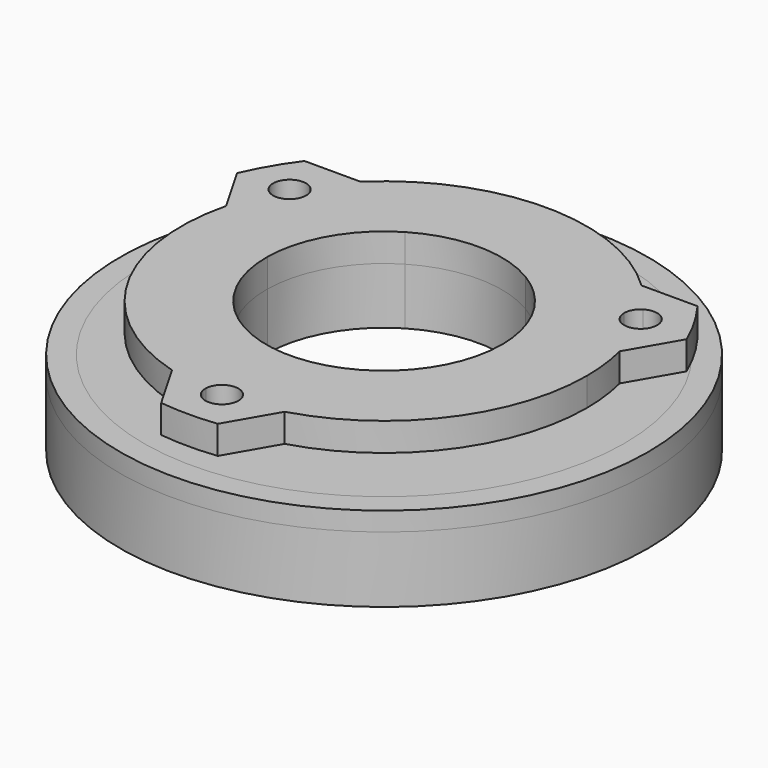
from build123d import *

# Parameters (mm, degrees)
F0_R          = 8.75
F0_R_2        = 7.75
F1_DEPTH      = 2
F0_R_3        = 12.75
F2_DEPTH      = 1
F0_R_4        = 14
F3_DEPTH      = 3.5
F3_DEPTH_BACK = 1
F5_DEPTH      = 1.5
F6_DEPTH      = 3


# Not quite as in the source:
# - ends of sketch curves that miss each other by under 0.0002 mm in the source are joined


with BuildPart() as f1:
    # F0 (on Top) → F1 (new body)
    with BuildSketch(Plane.XY):
        Circle(F0_R)
        Circle(F0_R_2, mode=Mode.SUBTRACT)
    extrude(amount=F1_DEPTH)

    # F0 (on Top) → F2 (join)
    with BuildSketch(Plane.XY):
        Circle(F0_R_3)
        Circle(F0_R, mode=Mode.SUBTRACT)
    extrude(amount=F2_DEPTH)

    # F0 (on Top) → F3 (join, two sides)
    with BuildSketch(Plane.XY) as f3_sk:
        Circle(F0_R_4)
        Circle(F0_R_3, mode=Mode.SUBTRACT)
    extrude(amount=-F3_DEPTH)
    extrude(f3_sk.sketch, amount=F3_DEPTH_BACK)


with BuildPart() as f5:
    # F4 (on face) → F5 (new body)
    with BuildSketch(Plane.XY.offset(2)):
        with BuildLine():
            Line((-7.4498323446, 7.7499998733), (-10.4241976301, 7.7499998733))
            ThreePointArc((-10.4241976301, 7.7499998733), (-11.2492131147, 6.49473622), (-11.9237955847, 5.1526200251))
            Line((-11.9237955847, 5.1526200251), (-10.436612942, 2.5767441277))
            ThreePointArc((-10.436612942, 2.5767441277), (-10.1269990673, 3.606437285), (-9.7160710573, 4.6000503485))
            ThreePointArc((-9.7160710573, 4.6000503485), (-10.067545319, 5.8125), (-8.8417959892, 6.1143391863))
            ThreePointArc((-8.8417959892, 6.1143391863), (-8.1867658396, 6.9670198139), (-7.4498323446, 7.7499998733))
        make_face()
        with BuildLine():
            Line((1.4995979546, -12.9026198984), (2.9867805973, -10.3267440011))
            ThreePointArc((2.9867805973, -10.3267440011), (1.9402332277, -10.5734570989), (0.8742750681, -10.7143895349))
            ThreePointArc((0.8742750681, -10.7143895349), (0.8748187483, -10.7321910784), (0.875, -10.75))
            ThreePointArc((0.875, -10.75), (-0.0178089216, -11.6248187483), (-0.8742750681, -10.7143895349))
            ThreePointArc((-0.8742750681, -10.7143895349), (-1.9402332277, -10.5734570989), (-2.9867805973, -10.3267440011))
            Line((-2.9867805973, -10.3267440011), (-1.4995979546, -12.9026198984))
            ThreePointArc((-1.4995979546, -12.9026198984), (0, -12.9894724399), (1.4995979546, -12.9026198984))
        make_face()
        with BuildLine():
            ThreePointArc((9.7160710573, 4.6000503485), (10.1269990673, 3.606437285), (10.436612942, 2.5767441277))
            Line((10.436612942, 2.5767441277), (11.9237955847, 5.1526200251))
            ThreePointArc((11.9237955847, 5.1526200251), (11.2492131147, 6.49473622), (10.4241976301, 7.7499998733))
            Line((10.4241976301, 7.7499998733), (7.4498323446, 7.7499998733))
            ThreePointArc((7.4498323446, 7.7499998733), (8.1867658396, 6.9670198139), (8.8417959892, 6.1143391863))
            ThreePointArc((8.8417959892, 6.1143391863), (9.7317594863, 6.1415197205), (10.1847730907, 5.375))
            ThreePointArc((10.1847730907, 5.375), (10.0584838896, 4.9221676474), (9.7160710573, 4.6000503485))
        make_face()
        with BuildLine():
            Line((4.062019444, 7.7499998733), (7.4498323446, 7.7499998733))
            ThreePointArc((7.4498323446, 7.7499998733), (0, 10.75), (-7.4498323446, 7.7499998733))
            Line((-7.4498323446, 7.7499998733), (-4.062019444, 7.7499998733))
            ThreePointArc((-4.062019444, 7.7499998733), (0, 8.75), (4.062019444, 7.7499998733))
        make_face()
        with BuildLine():
            Line((-4.062019444, 7.7499998733), (-7.4498323446, 7.7499998733))
            ThreePointArc((-7.4498323446, 7.7499998733), (-8.1867658396, 6.9670198139), (-8.8417959892, 6.1143391863))
            ThreePointArc((-8.8417959892, 6.1143391863), (-8.5432533702, 5.7969863956), (-8.4347730907, 5.375))
            Line((-8.4347730907, 5.375), (-6.9044822398, 5.375))
            ThreePointArc((-6.9044822398, 5.375), (-5.6103650411, 6.7146335794), (-4.062019444, 7.7499998733))
        make_face()
        with BuildLine():
            Line((-6.9044822398, 5.375), (-8.4347730907, 5.375))
            ThreePointArc((-8.4347730907, 5.375), (-8.5520008624, 4.9375), (-8.8722730907, 4.6172277717))
            Line((-8.8722730907, 4.6172277717), (-8.1071276653, 3.2919570197))
            ThreePointArc((-8.1071276653, 3.2919570197), (-7.5777222831, 4.375), (-6.9044822398, 5.375))
        make_face()
        with BuildLine():
            ThreePointArc((-9.7160710573, 4.6000503485), (-10.1269990673, 3.606437285), (-10.436612942, 2.5767441277))
            Line((-10.436612942, 2.5767441277), (-8.7427064916, -0.3571879075))
            ThreePointArc((-8.7427064916, -0.3571879075), (-8.6202257774, 1.5014018604), (-8.1071276653, 3.2919570197))
            Line((-8.1071276653, 3.2919570197), (-8.8722730907, 4.6172277717))
            ThreePointArc((-8.8722730907, 4.6172277717), (-9.2919641691, 4.5001812517), (-9.7160710573, 4.6000503485))
        make_face()
        with BuildLine():
            ThreePointArc((-10.436612942, 2.5767441277), (-9.3097730907, -5.375), (-2.9867805973, -10.3267440011))
            Line((-2.9867805973, -10.3267440011), (-4.6806870477, -7.3928119658))
            ThreePointArc((-4.6806870477, -7.3928119658), (-7.5777222831, -4.375), (-8.7427064916, -0.3571879075))
            Line((-8.7427064916, -0.3571879075), (-10.436612942, 2.5767441277))
        make_face()
        with BuildLine():
            ThreePointArc((-2.9867805973, -10.3267440011), (-1.9402332277, -10.5734570989), (-0.8742750681, -10.7143895349))
            ThreePointArc((-0.8742750681, -10.7143895349), (-0.7487107989, -10.2971676474), (-0.4375, -9.9922277717))
            Line((-0.4375, -9.9922277717), (-1.2026454254, -8.6669570197))
            ThreePointArc((-1.2026454254, -8.6669570197), (-3.0098607363, -8.2160354398), (-4.6806870477, -7.3928119658))
            Line((-4.6806870477, -7.3928119658), (-2.9867805973, -10.3267440011))
        make_face()
        with BuildLine():
            ThreePointArc((0.8742750681, -10.7143895349), (1.9402332277, -10.5734570989), (2.9867805973, -10.3267440011))
            Line((2.9867805973, -10.3267440011), (4.6806870477, -7.3928119658))
            ThreePointArc((4.6806870477, -7.3928119658), (3.0098607363, -8.2160354398), (1.2026454254, -8.6669570197))
            Line((1.2026454254, -8.6669570197), (0.4375, -9.9922277717))
            ThreePointArc((0.4375, -9.9922277717), (0.7487107989, -10.2971676474), (0.8742750681, -10.7143895349))
        make_face()
        with BuildLine():
            ThreePointArc((2.9867805973, -10.3267440011), (8.592740873, -6.4596675061), (10.75, 0))
            ThreePointArc((10.75, 0), (10.6713656372, 1.2978657238), (10.436612942, 2.5767441277))
            Line((10.436612942, 2.5767441277), (8.7427064916, -0.3571879075))
            ThreePointArc((8.7427064916, -0.3571879075), (7.5777222831, -4.375), (4.6806870477, -7.3928119658))
            Line((4.6806870477, -7.3928119658), (2.9867805973, -10.3267440011))
        make_face()
        with BuildLine():
            Line((8.7427064916, -0.3571879075), (10.436612942, 2.5767441277))
            ThreePointArc((10.436612942, 2.5767441277), (10.1269990673, 3.606437285), (9.7160710573, 4.6000503485))
            ThreePointArc((9.7160710573, 4.6000503485), (9.2919641691, 4.5001812517), (8.8722730907, 4.6172277717))
            Line((8.8722730907, 4.6172277717), (8.1071276653, 3.2919570197))
            ThreePointArc((8.1071276653, 3.2919570197), (8.5877781489, 1.6770707989), (8.75, 0))
            ThreePointArc((8.75, 0), (8.7481764329, -0.1786311819), (8.7427064916, -0.3571879075))
        make_face()
        with BuildLine():
            Line((8.1071276653, 3.2919570197), (8.8722730907, 4.6172277717))
            ThreePointArc((8.8722730907, 4.6172277717), (8.5520008624, 4.9375), (8.4347730907, 5.375))
            Line((8.4347730907, 5.375), (6.9044822398, 5.375))
            ThreePointArc((6.9044822398, 5.375), (7.5777222831, 4.375), (8.1071276653, 3.2919570197))
        make_face()
        with BuildLine():
            ThreePointArc((8.4347730907, 5.375), (8.5432533702, 5.7969863956), (8.8417959892, 6.1143391863))
            ThreePointArc((8.8417959892, 6.1143391863), (8.1867658396, 6.9670198139), (7.4498323446, 7.7499998733))
            Line((7.4498323446, 7.7499998733), (4.062019444, 7.7499998733))
            ThreePointArc((4.062019444, 7.7499998733), (5.6103650411, 6.7146335794), (6.9044822398, 5.375))
            Line((6.9044822398, 5.375), (8.4347730907, 5.375))
        make_face()
        with BuildLine():
            ThreePointArc((-0.4375, -9.9922277717), (0, -9.875), (0.4375, -9.9922277717))
            Line((0.4375, -9.9922277717), (1.2026454254, -8.6669570197))
            ThreePointArc((1.2026454254, -8.6669570197), (0, -8.75), (-1.2026454254, -8.6669570197))
            Line((-1.2026454254, -8.6669570197), (-0.4375, -9.9922277717))
        make_face()
        with BuildLine():
            Line((0, 7.7499998733), (4.062019444, 7.7499998733))
            ThreePointArc((4.062019444, 7.7499998733), (0, 8.75), (-4.062019444, 7.7499998733))
            Line((-4.062019444, 7.7499998733), (0, 7.7499998733))
        make_face()
        with BuildLine():
            Line((0, 7.7499998733), (-4.062019444, 7.7499998733))
            ThreePointArc((-4.062019444, 7.7499998733), (-5.6103650411, 6.7146335794), (-6.9044822398, 5.375))
            Line((-6.9044822398, 5.375), (-5.5831778585, 5.375))
            ThreePointArc((-5.5831778585, 5.375), (-3.0336652749, 7.1315759128), (0, 7.7499998733))
        make_face()
        with BuildLine():
            Line((-5.5831778585, 5.375), (-6.9044822398, 5.375))
            ThreePointArc((-6.9044822398, 5.375), (-7.5777222831, 4.375), (-8.1071276653, 3.2919570197))
            Line((-8.1071276653, 3.2919570197), (-7.4464754746, 2.1476738593))
            ThreePointArc((-7.4464754746, 2.1476738593), (-6.7116968793, 3.875), (-5.5831778585, 5.375))
        make_face()
        with BuildLine():
            Line((-8.7427064916, -0.3571879075), (-6.7116967696, -3.8749999367))
            ThreePointArc((-6.7116967696, -3.8749999367), (-7.6929585469, -0.9385567618), (-7.4464754746, 2.1476738593))
            Line((-7.4464754746, 2.1476738593), (-8.1071276653, 3.2919570197))
            ThreePointArc((-8.1071276653, 3.2919570197), (-8.6202257774, 1.5014018604), (-8.7427064916, -0.3571879075))
        make_face()
        with BuildLine():
            ThreePointArc((-8.7427064916, -0.3571879075), (-7.5777222831, -4.375), (-4.6806870477, -7.3928119658))
            Line((-4.6806870477, -7.3928119658), (-6.7116967696, -3.8749999367))
            Line((-6.7116967696, -3.8749999367), (-8.7427064916, -0.3571879075))
        make_face()
        with BuildLine():
            ThreePointArc((-4.6806870477, -7.3928119658), (-3.0098607363, -8.2160354398), (-1.2026454254, -8.6669570197))
            Line((-1.2026454254, -8.6669570197), (-1.8632976161, -7.5226738593))
            ThreePointArc((-1.8632976161, -7.5226738593), (-4.6592932721, -6.193019151), (-6.7116968793, -3.875))
            Line((-6.7116968793, -3.875), (-4.6806870477, -7.3928119658))
        make_face()
        with BuildLine():
            ThreePointArc((-1.2026454254, -8.6669570197), (0, -8.75), (1.2026454254, -8.6669570197))
            Line((1.2026454254, -8.6669570197), (1.8632976161, -7.5226738593))
            ThreePointArc((1.8632976161, -7.5226738593), (0, -7.75), (-1.8632976161, -7.5226738593))
            Line((-1.8632976161, -7.5226738593), (-1.2026454254, -8.6669570197))
        make_face()
        with BuildLine():
            ThreePointArc((1.2026454254, -8.6669570197), (3.0098607363, -8.2160354398), (4.6806870477, -7.3928119658))
            Line((4.6806870477, -7.3928119658), (6.7116967696, -3.8749999367))
            ThreePointArc((6.7116967696, -3.8749999367), (4.6592932721, -6.193019151), (1.8632976161, -7.5226738593))
            Line((1.8632976161, -7.5226738593), (1.2026454254, -8.6669570197))
        make_face()
        with BuildLine():
            ThreePointArc((4.6806870477, -7.3928119658), (7.5777222831, -4.375), (8.7427064916, -0.3571879075))
            Line((8.7427064916, -0.3571879075), (6.7116967696, -3.8749999367))
            Line((6.7116967696, -3.8749999367), (4.6806870477, -7.3928119658))
        make_face()
        with BuildLine():
            Line((6.7116967696, -3.8749999367), (8.7427064916, -0.3571879075))
            ThreePointArc((8.7427064916, -0.3571879075), (8.7481764329, -0.1786311819), (8.75, 0))
            ThreePointArc((8.75, 0), (8.5877781489, 1.6770707989), (8.1071276653, 3.2919570197))
            Line((8.1071276653, 3.2919570197), (7.4464754746, 2.1476738593))
            ThreePointArc((7.4464754746, 2.1476738593), (7.6737437059, 1.0845079695), (7.75, 0))
            ThreePointArc((7.75, 0), (7.4859251537, -2.0058475995), (6.7116967696, -3.8749999367))
        make_face()
        with BuildLine():
            Line((7.4464754746, 2.1476738593), (8.1071276653, 3.2919570197))
            ThreePointArc((8.1071276653, 3.2919570197), (7.5777222831, 4.375), (6.9044822398, 5.375))
            Line((6.9044822398, 5.375), (5.5831778585, 5.375))
            ThreePointArc((5.5831778585, 5.375), (6.7116968793, 3.875), (7.4464754746, 2.1476738593))
        make_face()
        with BuildLine():
            Line((5.5831778585, 5.375), (6.9044822398, 5.375))
            ThreePointArc((6.9044822398, 5.375), (5.6103650411, 6.7146335794), (4.062019444, 7.7499998733))
            Line((4.062019444, 7.7499998733), (0, 7.7499998733))
            ThreePointArc((0, 7.7499998733), (3.0336652749, 7.1315759128), (5.5831778585, 5.375))
        make_face()
        with BuildLine():
            Line((3.1893377055, 5.375), (5.5831778585, 5.375))
            ThreePointArc((5.5831778585, 5.375), (3.0336652749, 7.1315759128), (0, 7.75))
            ThreePointArc((0, 7.75), (-3.0336652749, 7.1315759128), (-5.5831778585, 5.375))
            Line((-5.5831778585, 5.375), (-3.1893377055, 5.375))
            ThreePointArc((-3.1893377055, 5.375), (0, 6.25), (3.1893377055, 5.375))
        make_face()
        with BuildLine():
            Line((-3.1893377055, 5.375), (-5.5831778585, 5.375))
            ThreePointArc((-5.5831778585, 5.375), (-6.7116968793, 3.875), (-7.4464754746, 2.1476738593))
            Line((-7.4464754746, 2.1476738593), (-6.2495553981, 0.0745474742))
            ThreePointArc((-6.2495553981, 0.0745474742), (-5.4126587737, 3.125), (-3.1893377055, 5.375))
        make_face()
        with BuildLine():
            ThreePointArc((-6.7116968793, -3.875), (-4.6592932721, -6.193019151), (-1.8632976161, -7.5226738593))
            Line((-1.8632976161, -7.5226738593), (-3.0602176926, -5.4495474742))
            ThreePointArc((-3.0602176926, -5.4495474742), (-5.4126587737, -3.125), (-6.2495553981, 0.0745474742))
            Line((-6.2495553981, 0.0745474742), (-7.4464754746, 2.1476738593))
            ThreePointArc((-7.4464754746, 2.1476738593), (-7.6929585469, -0.9385567618), (-6.7116968793, -3.875))
        make_face()
        with BuildLine():
            ThreePointArc((1.8632976161, -7.5226738593), (4.6592932721, -6.193019151), (6.7116968793, -3.875))
            ThreePointArc((6.7116968793, -3.875), (7.4859251537, -2.0058475995), (7.75, 0))
            ThreePointArc((7.75, 0), (7.6737437059, 1.0845079695), (7.4464754746, 2.1476738593))
            Line((7.4464754746, 2.1476738593), (6.2495553981, 0.0745474742))
            ThreePointArc((6.2495553981, 0.0745474742), (6.2498888485, 0.0372744), (6.25, 0))
            ThreePointArc((6.25, 0), (5.3939253137, -3.1572250016), (3.0602176926, -5.4495474742))
            Line((3.0602176926, -5.4495474742), (1.8632976161, -7.5226738593))
        make_face()
        with BuildLine():
            Line((6.2495553981, 0.0745474742), (7.4464754746, 2.1476738593))
            ThreePointArc((7.4464754746, 2.1476738593), (6.7116968793, 3.875), (5.5831778585, 5.375))
            Line((5.5831778585, 5.375), (3.1893377055, 5.375))
            ThreePointArc((3.1893377055, 5.375), (5.4126587737, 3.125), (6.2495553981, 0.0745474742))
        make_face()
        with BuildLine():
            ThreePointArc((-1.8632976161, -7.5226738593), (0, -7.75), (1.8632976161, -7.5226738593))
            Line((1.8632976161, -7.5226738593), (3.0602176926, -5.4495474742))
            ThreePointArc((3.0602176926, -5.4495474742), (0, -6.25), (-3.0602176926, -5.4495474742))
            Line((-3.0602176926, -5.4495474742), (-1.8632976161, -7.5226738593))
        make_face()
    extrude(amount=F5_DEPTH)

    # F4 (on face) → F6 (join)
    with BuildSketch(Plane.XY.offset(2)):
        with BuildLine():
            Line((3.1893377055, 5.375), (5.5831778585, 5.375))
            ThreePointArc((5.5831778585, 5.375), (3.0336652749, 7.1315759128), (0, 7.75))
            ThreePointArc((0, 7.75), (-3.0336652749, 7.1315759128), (-5.5831778585, 5.375))
            Line((-5.5831778585, 5.375), (-3.1893377055, 5.375))
            ThreePointArc((-3.1893377055, 5.375), (0, 6.25), (3.1893377055, 5.375))
        make_face()
        with BuildLine():
            Line((-3.1893377055, 5.375), (-5.5831778585, 5.375))
            ThreePointArc((-5.5831778585, 5.375), (-6.7116968793, 3.875), (-7.4464754746, 2.1476738593))
            Line((-7.4464754746, 2.1476738593), (-6.2495553981, 0.0745474742))
            ThreePointArc((-6.2495553981, 0.0745474742), (-5.4126587737, 3.125), (-3.1893377055, 5.375))
        make_face()
        with BuildLine():
            ThreePointArc((-6.7116968793, -3.875), (-4.6592932721, -6.193019151), (-1.8632976161, -7.5226738593))
            Line((-1.8632976161, -7.5226738593), (-3.0602176926, -5.4495474742))
            ThreePointArc((-3.0602176926, -5.4495474742), (-5.4126587737, -3.125), (-6.2495553981, 0.0745474742))
            Line((-6.2495553981, 0.0745474742), (-7.4464754746, 2.1476738593))
            ThreePointArc((-7.4464754746, 2.1476738593), (-7.6929585469, -0.9385567618), (-6.7116968793, -3.875))
        make_face()
        with BuildLine():
            ThreePointArc((-1.8632976161, -7.5226738593), (0, -7.75), (1.8632976161, -7.5226738593))
            Line((1.8632976161, -7.5226738593), (3.0602176926, -5.4495474742))
            ThreePointArc((3.0602176926, -5.4495474742), (0, -6.25), (-3.0602176926, -5.4495474742))
            Line((-3.0602176926, -5.4495474742), (-1.8632976161, -7.5226738593))
        make_face()
        with BuildLine():
            ThreePointArc((1.8632976161, -7.5226738593), (4.6592932721, -6.193019151), (6.7116968793, -3.875))
            ThreePointArc((6.7116968793, -3.875), (7.4859251537, -2.0058475995), (7.75, 0))
            ThreePointArc((7.75, 0), (7.6737437059, 1.0845079695), (7.4464754746, 2.1476738593))
            Line((7.4464754746, 2.1476738593), (6.2495553981, 0.0745474742))
            ThreePointArc((6.2495553981, 0.0745474742), (6.2498888485, 0.0372744), (6.25, 0))
            ThreePointArc((6.25, 0), (5.3939253137, -3.1572250016), (3.0602176926, -5.4495474742))
            Line((3.0602176926, -5.4495474742), (1.8632976161, -7.5226738593))
        make_face()
        with BuildLine():
            Line((6.2495553981, 0.0745474742), (7.4464754746, 2.1476738593))
            ThreePointArc((7.4464754746, 2.1476738593), (6.7116968793, 3.875), (5.5831778585, 5.375))
            Line((5.5831778585, 5.375), (3.1893377055, 5.375))
            ThreePointArc((3.1893377055, 5.375), (5.4126587737, 3.125), (6.2495553981, 0.0745474742))
        make_face()
    extrude(amount=-F6_DEPTH)


solid = Compound([f1.part, f5.part])
